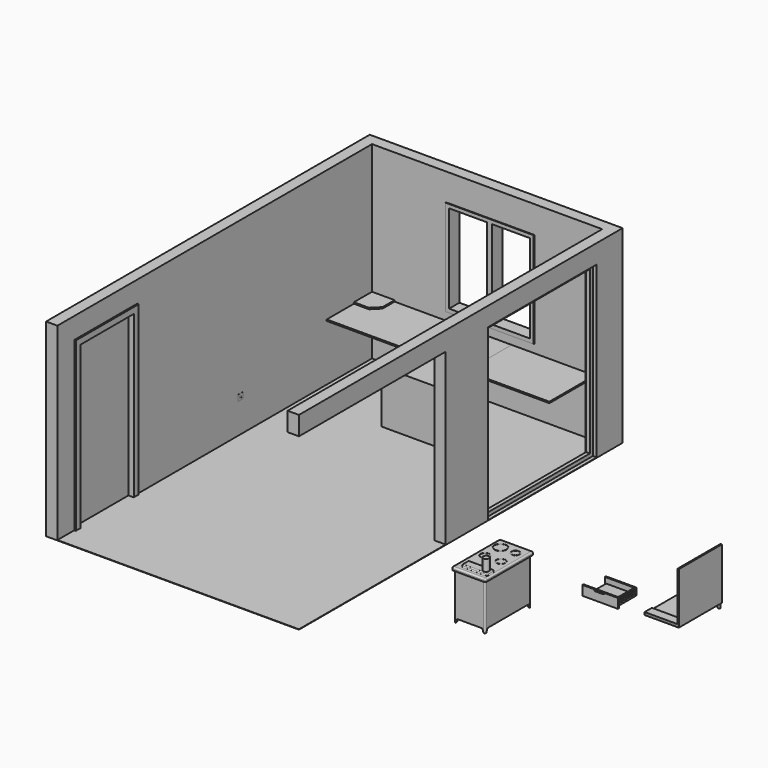
from build123d import *

# Parameters (mm, degrees)
F2_DEPTH       = 2500
F3_W           = 3350
F3_H           = 5360
F4_DEPTH       = 5
F6_START       = -50
F5_W           = 900
F5_H           = 2150
F6_DEPTH       = 50
F7_W           = 900
F7_H           = 350
F8_DEPTH       = 150
F10_DEPTH      = 20
F10_DEPTH_BACK = 170
F11_W          = 1170
F11_H          = 1270
F12_DEPTH      = 150
F13_W          = 1170
F13_H          = 1270
F13_W_2        = 500
F13_H_2        = 1170
F14_DEPTH      = 10
F14_DEPTH_BACK = 160
F15_W          = 80
F15_H          = 80
F15_R          = 17.8472983582
F16_DEPTH      = 1
F18_START      = 742
F17_W          = 1100
F17_H          = 750
F18_DEPTH      = 18
F20_START      = 742
F19_W          = 750
F19_H          = 750
F20_DEPTH      = 18
F22_START      = 742
F21_W          = 1100
F21_H          = 750
F22_DEPTH      = 18
F23_W          = 750
F23_H          = 470
F24_DEPTH      = 700
F25_W          = 434
F25_H          = 664
F25_W_2        = 426
F25_H_2        = 105.1666666667
F26_DEPTH      = 25
F27_W          = 434
F27_H          = 664
F27_W_2        = 426
F27_H_2        = 105.1666666667
F28_DEPTH      = 25
F30_DEPTH      = 18
F31_W          = 372
F31_H          = 315
F32_DEPTH      = 18
F33_W          = 315
F33_H          = 90
F34_DEPTH      = 18
F35_W          = 408
F35_H          = 90
F36_DEPTH      = 18
F37_W          = 470
F37_H          = 127
F38_DEPTH      = 18
F39_W          = 300
F39_H          = 36
F40_DEPTH      = 13
F42_DEPTH      = 9
F43_R          = 25
F44_R          = 1
F45_W          = 434
F45_H          = 714
F46_DEPTH      = 18
F47_W          = 714
F47_H          = 682
F48_DEPTH      = 18
F49_W          = 434
F49_H          = 120
F50_DEPTH      = 18
F51_W          = 42
F51_H          = 42
F52_DEPTH      = 2
F53_R          = 15
F54_DEPTH      = 58
F55_R          = 3
F56_W          = 300
F56_H          = 30
F57_DEPTH      = 10
F58_R          = 5
F59_W          = 450
F59_H          = 800
F60_DEPTH      = 650
F61_W          = 800
F61_H          = 611.0877394676
F62_DEPTH      = 20
F63_W          = 430
F63_H          = 611.0877394676
F64_DEPTH      = 20
F65_W          = 780
F65_H          = 625.4850495607
F66_DEPTH      = 20
F67_W          = 410
F67_H          = 611.0877394676
F68_DEPTH      = 20
F69_R          = 20
F70_R          = 83.4708998855
F70_R_2        = 74.1640641141
F70_R_3        = 56.7270025311
F70_R_4        = 48.1607857655
F70_R_5        = 61.9977401924
F70_R_6        = 53.4129503366
F70_R_7        = 61.2163146009
F70_R_8        = 52.8466902338
F71_DEPTH      = 3
F72_W          = 337.2278213501
F72_H          = 114.1590960324
F73_DEPTH      = 25
F74_R          = 12.49999
F75_R          = 38.110115234
F76_DEPTH      = 150
F77_W          = 293.0546998978
F77_H          = 200.7055580616
F77_W_2        = 249.6590092778
F77_H_2        = 83.7299227715
F78_DEPTH      = 10
F80_DEPTH      = 50
F80_TAPER      = 20
F81_W          = 150
F81_H          = 4930
F82_DEPTH      = 250
F83_W          = 150
F83_H          = 700
F84_DEPTH      = 2250
F86_START      = -50
F85_W          = 1800
F85_H          = 2250
F85_W_2        = 1700
F85_H_2        = 2150
F86_DEPTH      = 50


# Not quite as in the source:
# - a fillet or chamfer is up to 0.001 mm smaller than in the source, because OpenCascade refuses the exact size


with BuildPart() as f2:
    # F1 (on face) → F2 (new body)
    with BuildSketch(Plane.XY):
        Polygon((-278.3198941126, 4035.4139080613), (-278.3198941126, -74.5860919387), (-128.3198941126, -74.5860919387), (-128.3198941126, 3885.4139080613), (2921.6801058874, 3885.4139080613), (2921.6801058874, 3605.4139080613), (3071.6801058874, 3605.4139080613), (3071.6801058874, 3885.4139080613), (3071.6801058874, 4035.4139080613), (-128.3198941126, 4035.4139080613), align=None)
    extrude(amount=F2_DEPTH)

    # F7 (on face) → F8 (join, through all)
    with BuildSketch(Plane(origin=(-278.3198941126, 0, 0), x_dir=(0, -1, 0), z_dir=(-1, 0, 0))):
        with Locations((524.5860919387, 2325)):
            Rectangle(F7_W, F7_H)
        Polygon((974.5860919387, 2500), (974.5860919387, 2150), (974.5860919387, 0), (1324.5860919387, 0), (1324.5860919387, 2500), align=None)
    extrude(amount=-F8_DEPTH)

    # F11 (on face) → F12 (cut)
    with BuildSketch(Plane.XZ.offset(-3885.4139080613)):
        with Locations((1436.6801058874, 1505)):
            Rectangle(F11_W, F11_H)
    extrude(amount=-F12_DEPTH, mode=Mode.SUBTRACT)

    # F81 (on face) → F82 (join)
    with BuildSketch(Plane.XY.offset(2500)):
        with Locations((2996.6801058874, 1140.4139080613)):
            Rectangle(F81_W, F81_H)
    extrude(amount=-F82_DEPTH)

    # F83 (on face) → F84 (join, through all)
    with BuildSketch(Plane(origin=(0, 0, 2250), x_dir=(1, 0, 0), z_dir=(0, 0, -1))):
        with Locations((2996.6801058874, -1455.4139080613)):
            Rectangle(F83_W, F83_H)
    extrude(amount=F84_DEPTH)


with BuildPart() as f4:
    # F3 (on face) → F4 (new body)
    with BuildSketch(Plane(origin=(0, 0, 0), x_dir=(1, 0, 0), z_dir=(0, 0, -1))):
        with Locations((1396.6801058874, -1355.4139080613)):
            Rectangle(F3_W, F3_H)
    extrude(amount=F4_DEPTH)


with BuildPart() as f6:
    # F5 (on face) → F6 (new body)
    with BuildSketch(Plane(origin=(-278.3198941126, 0, 0), x_dir=(0, -1, 0), z_dir=(-1, 0, 0)).offset(F6_START)):
        with Locations((524.5860919387, 1075)):
            Rectangle(F5_W, F5_H)
    extrude(amount=-F6_DEPTH)


with BuildPart() as f10:
    # F9 (on face) → F10 (new body, two sides)
    with BuildSketch(Plane.YZ.offset(-128.3198941126)) as f10_sk:
        Polygon((-1044.5860919387, 2220), (-1044.5860919387, 0), (-964.5860919387, 0), (-964.5860919387, 2140), (-84.5860919387, 2140), (-84.5860919387, 0), (-4.5860919387, 0), (-4.5860919387, 2220), (-84.5860919387, 2220), (-964.5860919387, 2220), align=None)
    extrude(amount=F10_DEPTH)
    extrude(f10_sk.sketch, amount=-F10_DEPTH_BACK)


with BuildPart() as f14:
    # F13 (on face) → F14 (new body, two sides)
    with BuildSketch(Plane.XZ.offset(-3885.4139080613)) as f14_sk:
        with Locations((1436.6801058874, 1505)):
            Rectangle(F13_W, F13_H)
        with Locations((1151.6801058874, 1505)):
            Rectangle(F13_W_2, F13_H_2, mode=Mode.SUBTRACT)
        with Locations((1721.6801058874, 1505)):
            Rectangle(F13_W_2, F13_H_2, mode=Mode.SUBTRACT)
    extrude(amount=F14_DEPTH)
    extrude(f14_sk.sketch, amount=-F14_DEPTH_BACK)


with BuildPart() as f16:
    # F15 (on face) → F16 (new body)
    with BuildSketch(Plane.YZ.offset(-128.3198941126)):
        with Locations((1705.4139080613, 440)):
            Rectangle(F15_W, F15_H)
        with Locations((1705.4139080613, 440)):
            Circle(F15_R, mode=Mode.SUBTRACT)
    extrude(amount=F16_DEPTH)


with BuildPart() as f18:
    # F17 (on face) → F18 (new body)
    with BuildSketch(Plane.XY.offset(F18_START)):
        with Locations((421.6801058874, 3510.4139080613)):
            Rectangle(F17_W, F17_H)
    extrude(amount=F18_DEPTH)


with BuildPart() as f20:
    # F19 (on face) → F20 (new body)
    with BuildSketch(Plane.XY.offset(F20_START)):
        with Locations((1346.6801058874, 3510.4139080613)):
            Rectangle(F19_W, F19_H)
    extrude(amount=F20_DEPTH)


with BuildPart() as f22:
    # F21 (on face) → F22 (new body)
    with BuildSketch(Plane.XY.offset(F22_START)):
        with Locations((2271.6801058874, 3510.4139080613)):
            Rectangle(F21_W, F21_H)
    extrude(amount=F22_DEPTH)


with BuildPart() as f24:
    # F23 (on face) → F24 (new body)
    with BuildSketch(Plane.XY.offset(760)):
        with Locations((1346.6801058874, 2900.4139080613)):
            Rectangle(F23_W, F23_H)
    extrude(amount=-F24_DEPTH)

    # F25 (on face) → F26 (cut)
    with BuildSketch(Plane.YZ.offset(1721.6801058874)):
        with Locations((2900.4139080613, 410)):
            Rectangle(F25_W, F25_H)
        with Locations((2900.4139080613, 134.5833333333)):
            Rectangle(F25_W_2, F25_H_2, mode=Mode.SUBTRACT)
        with Locations((2900.4139080613, 244.75)):
            Rectangle(F25_W_2, F25_H_2, mode=Mode.SUBTRACT)
        with Locations((2900.4139080613, 354.9166666667)):
            Rectangle(F25_W_2, F25_H_2, mode=Mode.SUBTRACT)
        with Locations((2900.4139080613, 465.0833333333)):
            Rectangle(F25_W_2, F25_H_2, mode=Mode.SUBTRACT)
        with Locations((2900.4139080613, 575.25)):
            Rectangle(F25_W_2, F25_H_2, mode=Mode.SUBTRACT)
        with Locations((2900.4139080613, 685.4166666667)):
            Rectangle(F25_W_2, F25_H_2, mode=Mode.SUBTRACT)
    extrude(amount=-F26_DEPTH, mode=Mode.SUBTRACT)

    # F27 (on face) → F28 (cut)
    with BuildSketch(Plane(origin=(971.6801058874, 0, 0), x_dir=(0, -1, 0), z_dir=(-1, 0, 0))):
        with Locations((-2900.4139080613, 410)):
            Rectangle(F27_W, F27_H)
        with Locations((-2900.4139080613, 134.5833333333)):
            Rectangle(F27_W_2, F27_H_2, mode=Mode.SUBTRACT)
        with Locations((-2900.4139080613, 244.75)):
            Rectangle(F27_W_2, F27_H_2, mode=Mode.SUBTRACT)
        with Locations((-2900.4139080613, 354.9166666667)):
            Rectangle(F27_W_2, F27_H_2, mode=Mode.SUBTRACT)
        with Locations((-2900.4139080613, 465.0833333333)):
            Rectangle(F27_W_2, F27_H_2, mode=Mode.SUBTRACT)
        with Locations((-2900.4139080613, 575.25)):
            Rectangle(F27_W_2, F27_H_2, mode=Mode.SUBTRACT)
        with Locations((-2900.4139080613, 685.4166666667)):
            Rectangle(F27_W_2, F27_H_2, mode=Mode.SUBTRACT)
    extrude(amount=-F28_DEPTH, mode=Mode.SUBTRACT)


with BuildPart() as f30:
    # F29 (on face) → F30 (new body)
    with BuildSketch(Plane.XY.offset(760)):
        Polygon((171.6801058874, 3885.4139080613), (-128.3198941126, 3885.4139080613), (-128.3198941126, 3585.4139080613), (71.6801058874, 3585.4139080613), (171.6801058874, 3685.4139080613), align=None)
    extrude(amount=F30_DEPTH)


with BuildPart() as f32:
    # F31 (on Top) → F32 (new body)
    with BuildSketch(Plane.XY):
        with Locations((5122.1024990082, 1276.0291073359)):
            Rectangle(F31_W, F31_H)
    extrude(amount=F32_DEPTH)


with BuildPart() as f34:
    # F33 (on face) → F34 (new body)
    with BuildSketch(Plane.YZ.offset(5308.1024990082)):
        with Locations((1276.0291073359, 45)):
            Rectangle(F33_W, F33_H)
    extrude(amount=F34_DEPTH)


with BuildPart() as f36:
    # F35 (on face) → F36 (new body)
    with BuildSketch(Plane(origin=(0, 1433.5291073359, 0), x_dir=(-1, 0, 0), z_dir=(0, 1, 0))):
        with Locations((-5122.1024990082, 45)):
            Rectangle(F35_W, F35_H)
    extrude(amount=F36_DEPTH)


with BuildPart() as f38:
    # F37 (on face) → F38 (new body)
    with BuildSketch(Plane.XZ.offset(-1118.5291073359)):
        with Locations((5122.1024990082, 58.5)):
            Rectangle(F37_W, F37_H)
    extrude(amount=F38_DEPTH)


with BuildPart() as f40:
    # F39 (on face) → F40 (new body)
    with BuildSketch(Plane.YZ.offset(5326.1024990082)):
        with Locations((1276.1510968208, 53.8994505628)):
            Rectangle(F39_W, F39_H)
    extrude(amount=F40_DEPTH)

    # F56 (on face) → F57 (cut)
    with BuildSketch(Plane.YZ.offset(5339.1024990082)):
        with Locations((1276.1510968208, 53.8994505628)):
            Rectangle(F56_W, F56_H)
    extrude(amount=-F57_DEPTH, mode=Mode.SUBTRACT)

    # F58
    f58_edges = [f40.edges().sort_by_distance(p)[0] for p in [
        (5329.102499, 1276.151097, 38.899451),
        (5329.102499, 1276.151097, 68.899451),
        (5326.102499, 1276.151097, 35.899451),
        (5326.102499, 1276.151097, 71.899451),
    ]]
    fillet(f58_edges, radius=F58_R)


with BuildPart() as f42:
    # F41 (on face) → F42 (new body)
    with BuildSketch(Plane.XY.offset(122)):
        Polygon((5051.5582805776, 1100.5291073359), (5042.1024990082, 1100.5291073359), (5069.3469047546, 1070.5291073359), (5174.8580932617, 1070.5291073359), (5202.1024990082, 1100.5291073359), (5192.6467174388, 1100.5291073359), (5171.7593396998, 1077.5291073359), (5072.4456583165, 1077.5291073359), align=None)
    extrude(amount=F42_DEPTH)

    # F43
    f43_edges = [f42.edges().sort_by_distance(p)[0] for p in [
        (5069.346905, 1070.529107, 126.5),
        (5174.858093, 1070.529107, 126.5),
        (5072.445658, 1077.529107, 126.5),
        (5171.75934, 1077.529107, 126.5),
    ]]
    fillet(f43_edges, radius=F43_R)

    # F44
    f44_edges = [f42.edges().sort_by_distance(p)[0] for p in [
        (5052.004593, 1089.625482, 131),
        (5122.102499, 1070.529107, 131),
        (5122.102499, 1070.529107, 122),
        (5052.004593, 1089.625482, 122),
        (5192.200405, 1089.625482, 131),
        (5192.200405, 1089.625482, 122),
        (5185.923138, 1093.125482, 131),
        (5122.102499, 1077.529107, 131),
        (5058.28186, 1093.125482, 131),
        (5058.28186, 1093.125482, 122),
        (5122.102499, 1077.529107, 122),
        (5185.923138, 1093.125482, 122),
        (5170.812113, 1079.668866, 122),
        (5073.392885, 1079.668866, 122),
        (5173.910867, 1072.668866, 122),
        (5070.294131, 1072.668866, 122),
        (5170.812113, 1079.668866, 131),
        (5073.392885, 1079.668866, 131),
        (5173.910867, 1072.668866, 131),
        (5070.294131, 1072.668866, 131),
    ]]
    fillet(f44_edges, radius=F44_R)


with BuildPart() as f46:
    # F45 (on Top) → F46 (new body)
    with BuildSketch(Plane.XY):
        with Locations((5883.6476862937, 1514.6762795448)):
            Rectangle(F45_W, F45_H)
    extrude(amount=F46_DEPTH)


with BuildPart() as f48:
    # F47 (on face) → F48 (new body)
    with BuildSketch(Plane.YZ.offset(6100.6476862937)):
        with Locations((1514.6762795448, 341)):
            Rectangle(F47_W, F47_H)
    extrude(amount=F48_DEPTH)


with BuildPart() as f50:
    # F49 (on face) → F50 (new body)
    with BuildSketch(Plane.XY.offset(18)):
        with Locations((5883.6476862937, 1217.6762795448)):
            Rectangle(F49_W, F49_H)
    extrude(amount=F50_DEPTH)


with BuildPart() as f52:
    # F51 (on face) → F52 (new body)
    with BuildSketch(Plane(origin=(0, 0, 0), x_dir=(1, 0, 0), z_dir=(0, 0, -1))):
        with Locations((6097.6476862937, -1850.6762795448)):
            Rectangle(F51_W, F51_H)
    extrude(amount=F52_DEPTH)

    # F53 (on face) → F54 (join)
    with BuildSketch(Plane(origin=(0, 0, -2), x_dir=(1, 0, 0), z_dir=(0, 0, -1))):
        with Locations((6097.6476862937, -1850.6762795448)):
            Circle(F53_R)
    extrude(amount=F54_DEPTH)

    # F55
    f55_edges = [f52.edges().sort_by_distance(p)[0] for p in [
        (6082.647686, 1850.67628, -60),
    ]]
    fillet(f55_edges, radius=F55_R)


with BuildPart() as f60:
    # F59 (on Top) → F60 (new body)
    with BuildSketch(Plane.XY):
        with Locations((4432.626247406, 181.5961902235)):
            Rectangle(F59_W, F59_H)
    extrude(amount=F60_DEPTH)

    # F61 (on face) → F62 (cut)
    with BuildSketch(Plane.YZ.offset(4657.626247406)):
        with Locations((181.5961902235, 305.5438697338)):
            Rectangle(F61_W, F61_H)
    extrude(amount=-F62_DEPTH, mode=Mode.SUBTRACT)

    # F63 (on face) → F64 (cut)
    with BuildSketch(Plane.XZ.offset(218.4038097765)):
        with Locations((4422.626247406, 305.5438697338)):
            Rectangle(F63_W, F63_H)
    extrude(amount=-F64_DEPTH, mode=Mode.SUBTRACT)

    # F65 (on face) → F66 (cut)
    with BuildSketch(Plane(origin=(4207.626247406, 0, 0), x_dir=(0, -1, 0), z_dir=(-1, 0, 0))):
        with Locations((-191.5961902235, 298.3452146873)):
            Rectangle(F65_W, F65_H)
    extrude(amount=-F66_DEPTH, mode=Mode.SUBTRACT)

    # F67 (on face) → F68 (cut)
    with BuildSketch(Plane(origin=(0, 581.5961902235, 0), x_dir=(-1, 0, 0), z_dir=(0, 1, 0))):
        with Locations((-4432.626247406, 305.5438697338)):
            Rectangle(F67_W, F67_H)
    extrude(amount=-F68_DEPTH, mode=Mode.SUBTRACT)

    # F69
    f69_edges = [f60.edges().sort_by_distance(p)[0] for p in [
        (4432.626247, 581.59619, 650),
        (4207.626247, 181.59619, 650),
        (4432.626247, -218.40381, 650),
        (4657.626247, 181.59619, 650),
        (4657.626247, -218.40381, 630.54387),
        (4207.626247, -218.40381, 630.54387),
        (4207.626247, 581.59619, 630.54387),
        (4657.626247, 581.59619, 630.54387),
        (4637.626247, 561.59619, 305.54387),
        (4227.626247, 561.59619, 305.54387),
        (4227.626247, -198.40381, 305.54387),
        (4637.626247, -198.40381, 305.54387),
    ]]
    fillet(f69_edges, radius=F69_R)

    # F70 (on face) → F71 (cut)
    with BuildSketch(Plane.XY.offset(650)):
        with Locations((4336.2159729004, 432.3697090149)):
            Circle(F70_R)
        with Locations((4336.2159729004, 432.3697090149)):
            Circle(F70_R_2, mode=Mode.SUBTRACT)
        with Locations((4535.493850708, 432.3697090149)):
            Circle(F70_R_3)
        with Locations((4535.493850708, 432.3697090149)):
            Circle(F70_R_4, mode=Mode.SUBTRACT)
        with Locations((4325.2005577087, 191.0333931446)):
            Circle(F70_R_5)
        with Locations((4325.2005577087, 191.0333931446)):
            Circle(F70_R_6, mode=Mode.SUBTRACT)
        with Locations((4535.493850708, 191.0333931446)):
            Circle(F70_R_7)
        with Locations((4535.493850708, 191.0333931446)):
            Circle(F70_R_8, mode=Mode.SUBTRACT)
    extrude(amount=-F71_DEPTH, mode=Mode.SUBTRACT)

    # F72 (on face) → F73 (join)
    with BuildSketch(Plane.XY.offset(650)):
        with Locations((4456.4728736877, -92.1045150608)):
            Rectangle(F72_W, F72_H)
    extrude(amount=F73_DEPTH)

    # F74 (radius 12.5 in the source; OpenCascade refuses exactly that, so slightly less here)
    f74_edges = [f60.edges().sort_by_distance(p)[0] for p in [
        (4456.472874, -35.024967, 675),
        (4287.858963, -92.104515, 675),
        (4456.472874, -149.184063, 675),
        (4625.086784, -92.104515, 675),
        (4287.858963, -149.184063, 662.5),
        (4625.086784, -149.184063, 662.5),
        (4456.472874, -149.184063, 650),
        (4625.086784, -35.024967, 662.5),
        (4287.858963, -35.024967, 662.5),
        (4456.472874, -35.024967, 650),
        (4287.858963, -92.104515, 650),
        (4625.086784, -92.104515, 650),
    ]]
    fillet(f74_edges, radius=F74_R)

    # F75 (on face) → F76 (join)
    with BuildSketch(Plane.XY.offset(675)):
        with Locations((4567.7261352539, -93.7228053808)):
            Circle(F75_R)
    extrude(amount=F76_DEPTH)

    # F77 (on face) → F78 (join)
    with BuildSketch(Plane(origin=(4227.626247406, 0, 0), x_dir=(0, -1, 0), z_dir=(-1, 0, 0))):
        with Locations((-22.5176215172, 451.5496939421)):
            Rectangle(F77_W, F77_H)
        with Locations((-21.7522494495, 486.6423904896)):
            Rectangle(F77_W_2, F77_H_2, mode=Mode.SUBTRACT)
    extrude(amount=F78_DEPTH)

    # F79 (on face) → F80 (cut)
    with BuildSketch(Plane(origin=(0, 0, 0), x_dir=(1, 0, 0), z_dir=(0, 0, -1))):
        Polygon((4247.626247406, 178.4038097765), (4227.626247406, 178.4038097765), (4149.6381759644, 178.4038097765), (4149.6381759644, -541.5961902235), (4227.626247406, -541.5961902235), (4247.626247406, -541.5961902235), (4247.626247406, -561.5961902235), (4247.626247406, -663.2035970688), (4617.626247406, -663.2035970688), (4617.626247406, -561.5961902235), (4617.626247406, -541.5961902235), (4637.626247406, -541.5961902235), (4716.450214386, -541.5961902235), (4716.450214386, 178.4038097765), (4637.626247406, 178.4038097765), (4617.626247406, 178.4038097765), (4617.626247406, 304.9205813699), (4247.626247406, 304.9205813699), align=None)
    extrude(amount=-F80_DEPTH, taper=F80_TAPER, mode=Mode.SUBTRACT)


with BuildPart() as f86:
    # F85 (on face) → F86 (new body)
    with BuildSketch(Plane.YZ.offset(3071.6801058874).offset(F86_START)):
        with Locations((2705.4139080613, 1125)):
            Rectangle(F85_W, F85_H)
        with Locations((2705.4139080613, 1125)):
            Rectangle(F85_W_2, F85_H_2, mode=Mode.SUBTRACT)
    extrude(amount=-F86_DEPTH)


solid = Compound([f2.part, f4.part, f6.part, f10.part, f14.part, f16.part, f18.part, f20.part, f22.part, f24.part, f30.part, f32.part, f34.part, f36.part, f38.part, f40.part, f42.part, f46.part, f48.part, f50.part, f52.part, f60.part, f86.part])
